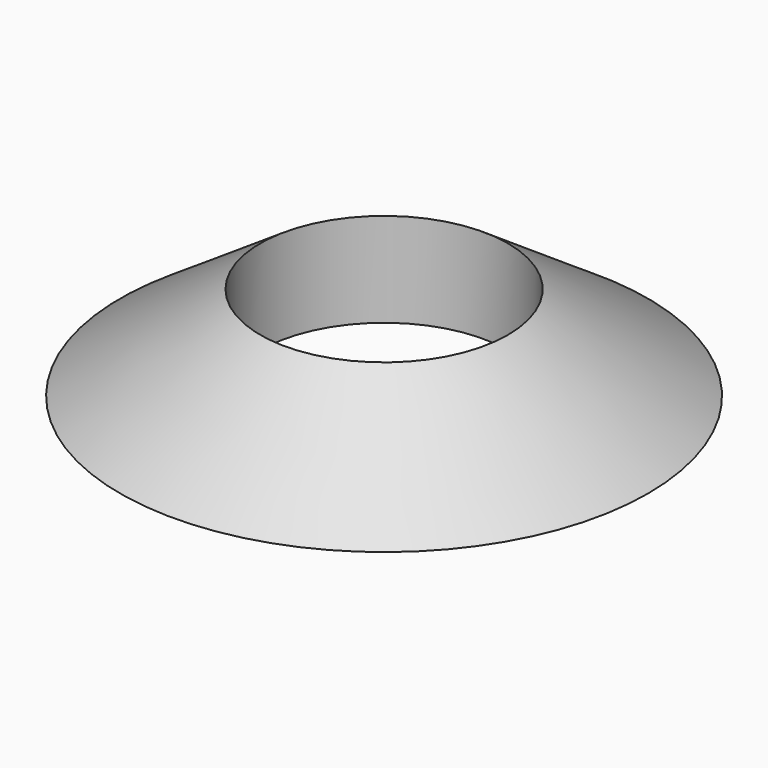
from build123d import *

# Parameters (mm, degrees)
F0_R     = 29.21
F2_R     = 13.7106345788
F6_R     = 13.7106345788
F7_DEPTH = 37.846


# Not quite as in the source:
# - the program builds the solid bodies; features that only make, move or delete a surface that nothing else refers to are left out


with BuildPart() as f3:
    # F0 (on Top) → F3 section 0
    with BuildSketch(Plane.XY):
        Circle(F0_R)
    # F2 (on offset) → F3 section 1
    with BuildSketch(Plane.XY.offset(10.414)):
        Circle(F2_R)
    loft()

    # F6 (on Top) → F7 (cut)
    with BuildSketch(Plane.XY):
        Circle(F6_R)
    extrude(amount=F7_DEPTH, mode=Mode.SUBTRACT)


solid = f3.part
